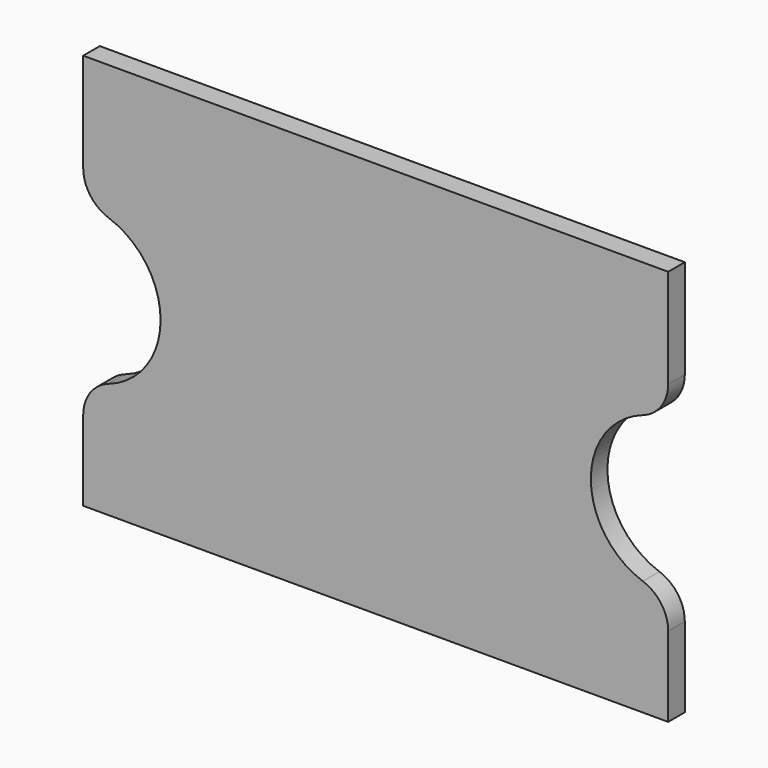
from build123d import *

# Parameters (mm, degrees)
F1_DEPTH = 2.2
F2_R     = 4


with BuildPart() as f1:
    # F0 (on Front) → F1 (new body)
    with BuildSketch(Plane.XZ):
        with BuildLine():
            Line((-31, 0), (31, 0))
            Line((31, 0), (31, 11.8))
            ThreePointArc((31, 11.8), (22.8, 20), (31, 28.2))
            Line((31, 28.2), (31, 42))
            Line((31, 42), (-31, 42))
            Line((-31, 42), (-31, 28.2))
            ThreePointArc((-31, 28.2), (-22.8, 20), (-31, 11.8))
            Line((-31, 11.8), (-31, 0))
        make_face()
    extrude(amount=F1_DEPTH)

    # F2
    f2_edges = [f1.edges().sort_by_distance(p)[0] for p in [
        (-31, -1.1, 11.8),
        (31, -1.1, 11.8),
        (31, -1.1, 28.2),
        (-31, -1.1, 28.2),
    ]]
    fillet(f2_edges, radius=F2_R)


solid = f1.part
